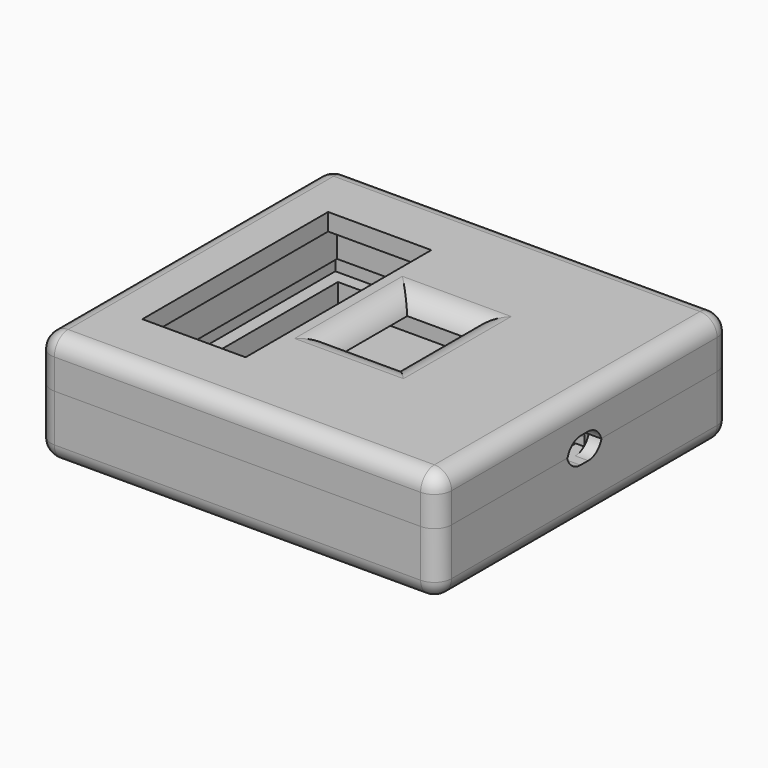
from build123d import *

# Parameters (mm, degrees)
F2_W          = 46.6
F2_H          = 42.6
F3_DEPTH      = 6
F5_W          = 37.6
F5_H          = 33.6
F6_DEPTH      = 4.5
F8_W          = 40.6
F8_H          = 36.6
F8_W_2        = 37.6
F8_H_2        = 33.6
F9_DEPTH      = 2
F10_W         = 46.6
F10_H         = 42.6
F10_W_2       = 43.6
F10_H_2       = 39.6
F11_DEPTH     = 1.5
F12_R         = 2
F13_W         = 1.5
F13_H         = 5
F14_DEPTH     = 1.5
F15_T1_DEPTH  = 1.5
F16_R         = 2
F18_W         = 46.6
F18_H         = 42.6
F19_DEPTH     = 7
F20_W         = 38.6
F20_H         = 34.6
F21_DEPTH     = 5
F22_W         = 46.6
F22_H         = 42.6
F22_W_2       = 42.6
F22_H_2       = 38.6
F23_DEPTH     = 1.5
F24_W         = 5
F24_H         = 5
F25_DEPTH     = 3
F26_T4_DEPTH  = 4
F26_T10_DEPTH = 4
F26_T16_DEPTH = 4
F26_T22_DEPTH = 4
F26_T28_DEPTH = 4
F26_T34_DEPTH = 4
F27_W         = 7
F27_H         = 10
F27_W_2       = 12
F27_H_2       = 27
F28_DEPTH     = 9.4
F29_R         = 2
F30_R         = 2
F31_T1_DEPTH  = 7
F31_T3_DEPTH  = 10
F31_T9_DEPTH  = 14.0710678119
F31_T14_DEPTH = 17.0710678119
F31_T21_DEPTH = 17.0710678119
F31_T25_DEPTH = 14.0710678119
F31_T32_DEPTH = 14.0710678119
F31_T36_DEPTH = 17.0710678119
F31_T43_DEPTH = 14.0710678119
F31_T48_DEPTH = 17.0710678119


# Not quite as in the source:
# - a fillet or chamfer that OpenCascade refuses, or shapes differently, is made with other operations: its cross-section is extruded or revolved along the edge and cut away or added


with BuildPart() as f3:
    # F2 (on Top) → F3 (new body)
    with BuildSketch(Plane.XY):
        Rectangle(F2_W, F2_H)
    extrude(amount=F3_DEPTH)

    # F5 (on offset) → F6 (cut)
    with BuildSketch(Plane.XY.offset(1.5)):
        Rectangle(F5_W, F5_H)
    extrude(amount=F6_DEPTH, mode=Mode.SUBTRACT)

    # F8 (on offset) → F9 (cut)
    with BuildSketch(Plane.XY.offset(4)):
        Rectangle(F8_W, F8_H)
        Rectangle(F8_W_2, F8_H_2, mode=Mode.SUBTRACT)
    extrude(amount=F9_DEPTH, mode=Mode.SUBTRACT)

    # F10 (on face) → F11 (join)
    with BuildSketch(Plane.XY.offset(6)):
        Rectangle(F10_W, F10_H)
        Rectangle(F10_W_2, F10_H_2, mode=Mode.SUBTRACT)
    extrude(amount=F11_DEPTH)

    # F12
    f12_edges = [f3.edges().sort_by_distance(p)[0] for p in [
        (-23.3, 21.3, 3.75),
        (-23.3, -21.3, 3.75),
        (23.3, 21.3, 3.75),
        (23.3, -21.3, 3.75),
    ]]
    fillet(f12_edges, radius=F12_R)

    # F13 (on face) → F14 (cut)
    with BuildSketch(Plane.XY.offset(7.5)):
        with Locations((22.55, 0)):
            Rectangle(F13_W, F13_H)
    extrude(amount=-F14_DEPTH, mode=Mode.SUBTRACT)

    # F15: fillet of radius 2 on 2 edges, made by hand

    # F15_s2 → F15_t1 (join)
    with BuildSketch(Plane.YZ.offset(21.8)):
        with BuildLine():
            ThreePointArc((-2.5, 7.5), (-1.7882531983, 6.4188611699), (-0.5635083269, 6))
            Line((-0.5635083269, 6), (-2.5, 6))
            Line((-2.5, 6), (-2.5, 7.5))
        make_face()
        with BuildLine():
            ThreePointArc((2.5, 7.5), (1.7882531983, 6.4188611699), (0.5635083269, 6))
            Line((0.5635083269, 6), (2.5, 6))
            Line((2.5, 6), (2.5, 7.5))
        make_face()
    extrude(amount=F15_T1_DEPTH)

    # F16
    f16_edges = [f3.edges().sort_by_distance(p)[0] for p in [
        (-23.3, 0, 0),
    ]]
    fillet(f16_edges, radius=F16_R)


with BuildPart() as f19:
    # F18 (on offset) → F19 (new body)
    with BuildSketch(Plane.XY.offset(6)):
        Rectangle(F18_W, F18_H)
    extrude(amount=F19_DEPTH)

    # F20 (on offset) → F21 (cut)
    with BuildSketch(Plane.XY.offset(6)):
        Rectangle(F20_W, F20_H)
    extrude(amount=F21_DEPTH, mode=Mode.SUBTRACT)

    # F22 (on face) → F23 (cut)
    with BuildSketch(Plane(origin=(0, 0, 6), x_dir=(1, 0, 0), z_dir=(0, 0, -1))):
        Rectangle(F22_W, F22_H)
        Rectangle(F22_W_2, F22_H_2, mode=Mode.SUBTRACT)
    extrude(amount=-F23_DEPTH, mode=Mode.SUBTRACT)

    # F24 (on offset) → F25 (cut)
    with BuildSketch(Plane.XY.offset(6)):
        with Locations((20.8, 0)):
            Rectangle(F24_W, F24_H)
    extrude(amount=F25_DEPTH, mode=Mode.SUBTRACT)

    # F26: fillet of radius 2 on 2 edges, made by hand


with BuildPart() as f26_tool2:
    # F26_s3 → F26_t4 (new body)
    with BuildSketch(Plane.YZ.offset(23.3)):
        with BuildLine():
            ThreePointArc((2.5, 7), (1.9142135624, 8.4142135624), (0.5, 9))
            Line((0.5, 9), (2.5, 9))
            Line((2.5, 9), (2.5, 7))
        make_face()
    extrude(amount=-F26_T4_DEPTH)

    split(bisect_by=Plane.XY.offset(7.5), keep=Keep.TOP)

    split(bisect_by=Plane.YZ.offset(21.3), keep=Keep.TOP)


with BuildPart() as f19_1:
    add(f19.part)

    # F26_t1: union F26_tool2
    add(f26_tool2.part)


with BuildPart() as f26_tool8:
    # F26_s9 → F26_t10 (new body)
    with BuildSketch(Plane.YZ.offset(23.3)):
        with BuildLine():
            ThreePointArc((2.5, 7), (1.9142135624, 8.4142135624), (0.5, 9))
            Line((0.5, 9), (2.5, 9))
            Line((2.5, 9), (2.5, 7))
        make_face()
    extrude(amount=-F26_T10_DEPTH)

    split(bisect_by=Plane.XY.offset(7.5), keep=Keep.BOTTOM)

    split(bisect_by=Plane.YZ.offset(21.3), keep=Keep.BOTTOM)


with BuildPart() as f19_2:
    add(f19_1.part)

    # F26_t7: union F26_tool8
    add(f26_tool8.part)


with BuildPart() as f26_tool14:
    # F26_s15 → F26_t16 (new body)
    with BuildSketch(Plane.YZ.offset(23.3)):
        with BuildLine():
            ThreePointArc((2.5, 7), (1.9142135624, 8.4142135624), (0.5, 9))
            Line((0.5, 9), (2.5, 9))
            Line((2.5, 9), (2.5, 7))
        make_face()
    extrude(amount=-F26_T16_DEPTH)

    split(bisect_by=Plane.XY.offset(7.5), keep=Keep.TOP)

    split(bisect_by=Plane.YZ.offset(21.3), keep=Keep.BOTTOM)


with BuildPart() as f19_3:
    add(f19_2.part)

    # F26_t13: union F26_tool14
    add(f26_tool14.part)


with BuildPart() as f26_tool20:
    # F26_s21 → F26_t22 (new body)
    with BuildSketch(Plane.YZ.offset(19.3)):
        with BuildLine():
            ThreePointArc((-2.5, 7), (-1.9142135624, 8.4142135624), (-0.5, 9))
            Line((-0.5, 9), (-2.5, 9))
            Line((-2.5, 9), (-2.5, 7))
        make_face()
    extrude(amount=F26_T22_DEPTH)

    split(bisect_by=Plane.XY.offset(7.5), keep=Keep.BOTTOM)

    split(bisect_by=Plane.YZ.offset(21.3), keep=Keep.BOTTOM)


with BuildPart() as f19_4:
    add(f19_3.part)

    # F26_t19: union F26_tool20
    add(f26_tool20.part)


with BuildPart() as f26_tool26:
    # F26_s27 → F26_t28 (new body)
    with BuildSketch(Plane.YZ.offset(19.3)):
        with BuildLine():
            ThreePointArc((-2.5, 7), (-1.9142135624, 8.4142135624), (-0.5, 9))
            Line((-0.5, 9), (-2.5, 9))
            Line((-2.5, 9), (-2.5, 7))
        make_face()
    extrude(amount=F26_T28_DEPTH)

    split(bisect_by=Plane.XY.offset(7.5), keep=Keep.TOP)

    split(bisect_by=Plane.YZ.offset(21.3), keep=Keep.BOTTOM)


with BuildPart() as f19_5:
    add(f19_4.part)

    # F26_t25: union F26_tool26
    add(f26_tool26.part)


with BuildPart() as f26_tool32:
    # F26_s33 → F26_t34 (new body)
    with BuildSketch(Plane.YZ.offset(19.3)):
        with BuildLine():
            ThreePointArc((-2.5, 7), (-1.9142135624, 8.4142135624), (-0.5, 9))
            Line((-0.5, 9), (-2.5, 9))
            Line((-2.5, 9), (-2.5, 7))
        make_face()
    extrude(amount=F26_T34_DEPTH)

    split(bisect_by=Plane.XY.offset(7.5), keep=Keep.TOP)

    split(bisect_by=Plane.YZ.offset(21.3), keep=Keep.TOP)


with BuildPart() as f19_6:
    add(f19_5.part)

    # F26_t31: union F26_tool32
    add(f26_tool32.part)

    # F27 (on offset) → F28 (cut)
    with BuildSketch(Plane.XY.offset(6)):
        with Locations((2.2, 0)):
            Rectangle(F27_W, F27_H)
        with Locations((-11.3, 0)):
            Rectangle(F27_W_2, F27_H_2)
    extrude(amount=F28_DEPTH, mode=Mode.SUBTRACT)

    # F29
    f29_edges = [f19_6.edges().sort_by_distance(p)[0] for p in [
        (-23.3, -21.3, 10.25),
        (23.3, -21.3, 10.25),
        (23.3, 21.3, 10.25),
        (-23.3, 21.3, 10.25),
    ]]
    fillet(f29_edges, radius=F29_R)

    # F30
    f30_edges = [f19_6.edges().sort_by_distance(p)[0] for p in [
        (23.3, 0, 13),
        (0, 21.3, 13),
        (-22.714214, 20.714214, 13),
        (22.714214, 20.714214, 13),
        (-23.3, 0, 13),
        (22.714214, -20.714214, 13),
        (-22.714214, -20.714214, 13),
        (0, -21.3, 13),
    ]]
    fillet(f30_edges, radius=F30_R)

    # F31: fillet of radius 3 on 4 edges, made by hand

    # F31_s2 → F31_t1 (cut)
    with BuildSketch(Plane.YZ.offset(-1.3)):
        with BuildLine():
            ThreePointArc((7.8284271247, 13), (6.0963763172, 12.4494897428), (5, 11))
            Line((5, 11), (5, 13))
            Line((5, 13), (7.8284271247, 13))
        make_face()
        with BuildLine():
            ThreePointArc((-7.8284271247, 13), (-6.0963763172, 12.4494897428), (-5, 11))
            Line((-5, 11), (-5, 13))
            Line((-5, 13), (-7.8284271247, 13))
        make_face()
    extrude(amount=F31_T1_DEPTH, mode=Mode.SUBTRACT)

    # F31_s4 → F31_t3 (cut)
    with BuildSketch(Plane.XZ.offset(-5)):
        with BuildLine():
            ThreePointArc((8.5284271247, 13), (6.7963763172, 12.4494897428), (5.7, 11))
            Line((5.7, 11), (5.7, 13))
            Line((5.7, 13), (8.5284271247, 13))
        make_face()
        with BuildLine():
            ThreePointArc((-4.1284271247, 13), (-2.3963763172, 12.4494897428), (-1.3, 11))
            Line((-1.3, 11), (-1.3, 13))
            Line((-1.3, 13), (-4.1284271247, 13))
        make_face()
    extrude(amount=F31_T3_DEPTH, mode=Mode.SUBTRACT)


with BuildPart() as f31_tool7:
    # F31_s8 → F31_t9 (new body)
    with BuildSketch(Plane.YZ.offset(-8.3710678119)):
        with BuildLine():
            ThreePointArc((7.8284271247, 13), (6.0963763172, 12.4494897428), (5, 11))
            Line((5, 11), (5, 13))
            Line((5, 13), (7.8284271247, 13))
        make_face()
    extrude(amount=F31_T9_DEPTH)

    split(bisect_by=Plane.YZ.offset(-5.3), keep=Keep.TOP)

    split(bisect_by=Plane.YZ.offset(-1.3), keep=Keep.BOTTOM)


with BuildPart() as f31_tool12:
    # F31_s13 → F31_t14 (new body)
    with BuildSketch(Plane.XZ.offset(5)):
        with BuildLine():
            ThreePointArc((-4.1284271247, 13), (-2.3963763172, 12.4494897428), (-1.3, 11))
            Line((-1.3, 11), (-1.3, 13))
            Line((-1.3, 13), (-4.1284271247, 13))
        make_face()
    extrude(amount=-F31_T14_DEPTH)

    split(bisect_by=Plane.XZ.offset(-5), keep=Keep.BOTTOM)


with BuildPart() as f31_tool7_1:
    add(f31_tool7.part)

    # F31_t16: intersect F31_tool12
    add(f31_tool12.part, mode=Mode.INTERSECT)


with BuildPart() as f19_7:
    add(f19_6.part)

    # F31_t5: cut F31_tool7
    add(f31_tool7_1.part, mode=Mode.SUBTRACT)


with BuildPart() as f31_tool19:
    # F31_s20 → F31_t21 (new body)
    with BuildSketch(Plane.XZ.offset(-12.0710678119)):
        with BuildLine():
            ThreePointArc((8.5284271247, 13), (6.7963763172, 12.4494897428), (5.7, 11))
            Line((5.7, 11), (5.7, 13))
            Line((5.7, 13), (8.5284271247, 13))
        make_face()
    extrude(amount=F31_T21_DEPTH)

    split(bisect_by=Plane.XZ.offset(-5), keep=Keep.BOTTOM)


with BuildPart() as f31_tool23:
    # F31_s24 → F31_t25 (new body)
    with BuildSketch(Plane.YZ.offset(-1.3)):
        with BuildLine():
            ThreePointArc((7.8284271247, 13), (6.0963763172, 12.4494897428), (5, 11))
            Line((5, 11), (5, 13))
            Line((5, 13), (7.8284271247, 13))
        make_face()
    extrude(amount=F31_T25_DEPTH)

    split(bisect_by=Plane.YZ.offset(5.7), keep=Keep.TOP)


with BuildPart() as f31_tool19_1:
    add(f31_tool19.part)

    # F31_t27: intersect F31_tool23
    add(f31_tool23.part, mode=Mode.INTERSECT)


with BuildPart() as f19_8:
    add(f19_7.part)

    # F31_t17: cut F31_tool19
    add(f31_tool19_1.part, mode=Mode.SUBTRACT)


with BuildPart() as f31_tool30:
    # F31_s31 → F31_t32 (new body)
    with BuildSketch(Plane.YZ.offset(12.7710678119)):
        with BuildLine():
            ThreePointArc((-7.8284271247, 13), (-6.0963763172, 12.4494897428), (-5, 11))
            Line((-5, 11), (-5, 13))
            Line((-5, 13), (-7.8284271247, 13))
        make_face()
    extrude(amount=-F31_T32_DEPTH)

    split(bisect_by=Plane.YZ.offset(5.7), keep=Keep.TOP)


with BuildPart() as f31_tool34:
    # F31_s35 → F31_t36 (new body)
    with BuildSketch(Plane.XZ.offset(-5)):
        with BuildLine():
            ThreePointArc((8.5284271247, 13), (6.7963763172, 12.4494897428), (5.7, 11))
            Line((5.7, 11), (5.7, 13))
            Line((5.7, 13), (8.5284271247, 13))
        make_face()
    extrude(amount=F31_T36_DEPTH)

    split(bisect_by=Plane.XZ.offset(5), keep=Keep.TOP)


with BuildPart() as f31_tool30_1:
    add(f31_tool30.part)

    # F31_t38: intersect F31_tool34
    add(f31_tool34.part, mode=Mode.INTERSECT)


with BuildPart() as f19_9:
    add(f19_8.part)

    # F31_t28: cut F31_tool30
    add(f31_tool30_1.part, mode=Mode.SUBTRACT)


with BuildPart() as f31_tool41:
    # F31_s42 → F31_t43 (new body)
    with BuildSketch(Plane.YZ.offset(5.7)):
        with BuildLine():
            ThreePointArc((-7.8284271247, 13), (-6.0963763172, 12.4494897428), (-5, 11))
            Line((-5, 11), (-5, 13))
            Line((-5, 13), (-7.8284271247, 13))
        make_face()
    extrude(amount=-F31_T43_DEPTH)

    split(bisect_by=Plane.YZ.offset(-5.3), keep=Keep.TOP)

    split(bisect_by=Plane.YZ.offset(-1.3), keep=Keep.BOTTOM)


with BuildPart() as f31_tool46:
    # F31_s47 → F31_t48 (new body)
    with BuildSketch(Plane.XZ.offset(12.0710678119)):
        with BuildLine():
            ThreePointArc((-4.1284271247, 13), (-2.3963763172, 12.4494897428), (-1.3, 11))
            Line((-1.3, 11), (-1.3, 13))
            Line((-1.3, 13), (-4.1284271247, 13))
        make_face()
    extrude(amount=-F31_T48_DEPTH)

    split(bisect_by=Plane.XZ.offset(5), keep=Keep.TOP)


with BuildPart() as f31_tool41_1:
    add(f31_tool41.part)

    # F31_t50: intersect F31_tool46
    add(f31_tool46.part, mode=Mode.INTERSECT)


with BuildPart() as f19_10:
    add(f19_9.part)

    # F31_t39: cut F31_tool41
    add(f31_tool41_1.part, mode=Mode.SUBTRACT)


solid = Compound([f3.part, f19_10.part])
